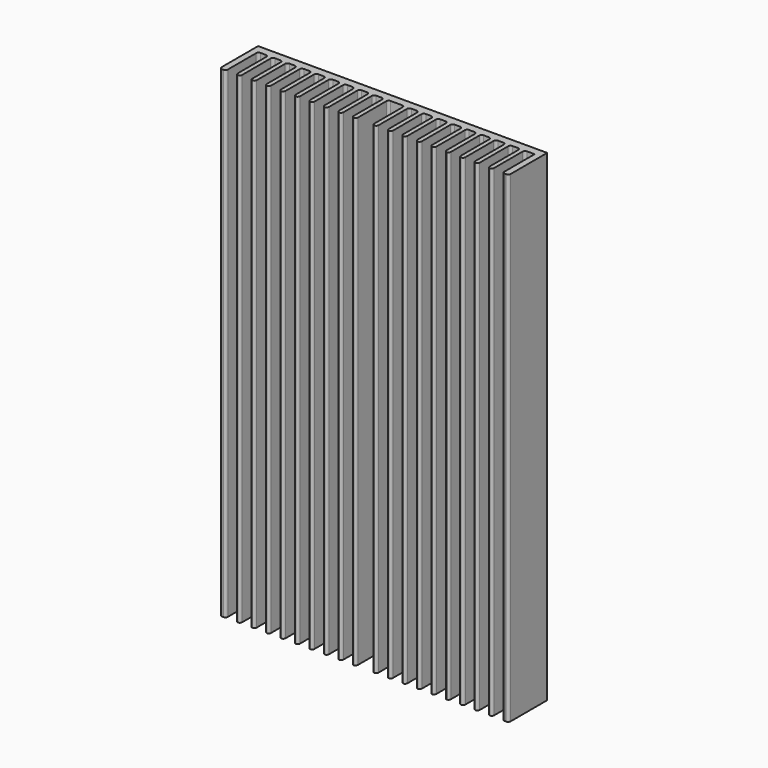
from build123d import *

# Parameters (mm, degrees)
F0_W        = 60
F0_H        = 100
F1_DEPTH    = 10
F2_W        = 2.0929928869
F2_H        = 8.3745439677
F2_W_2      = 1.2923884243
F2_W_3      = 0.8006044626
F3_DEPTH    = 100.001
F4_T1_DEPTH = 100
F4_T3_DEPTH = 102.5


# Not quite as in the source:
# - a fillet or chamfer that OpenCascade refuses, or shapes differently, is made with other operations: its cross-section is extruded or revolved along the edge and cut away or added


with BuildPart() as f1:
    # F0 (on Front) → F1 (new body)
    with BuildSketch(Plane.XZ):
        Rectangle(F0_W, F0_H)
    extrude(amount=F1_DEPTH)

    # F2 (on face) → F3 (cut, through all)
    with BuildSketch(Plane(origin=(0, 0, -50), x_dir=(1, 0, 0), z_dir=(0, 0, -1))):
        with Locations((-27.6461942121, 5.8127280162)):
            Rectangle(F2_W, F2_H)
        with Locations((-24.6461942121, 5.8127280162)):
            Rectangle(F2_W, F2_H)
        with Locations((-21.6461942121, 5.8127280162)):
            Rectangle(F2_W, F2_H)
        with Locations((27.6461942121, 5.8127280162)):
            Rectangle(F2_W, F2_H)
        with Locations((-18.6461942121, 5.8127280162)):
            Rectangle(F2_W, F2_H)
        with Locations((24.6461942121, 5.8127280162)):
            Rectangle(F2_W, F2_H)
        with Locations((-15.6461942121, 5.8127280162)):
            Rectangle(F2_W, F2_H)
        with Locations((21.6461942121, 5.8127280162)):
            Rectangle(F2_W, F2_H)
        with Locations((-12.6461942121, 5.8127280162)):
            Rectangle(F2_W, F2_H)
        with Locations((18.6461942121, 5.8127280162)):
            Rectangle(F2_W, F2_H)
        with Locations((-9.6461942121, 5.8127280162)):
            Rectangle(F2_W, F2_H)
        with Locations((15.6461942121, 5.8127280162)):
            Rectangle(F2_W, F2_H)
        with Locations((-6.6461942121, 5.8127280162)):
            Rectangle(F2_W, F2_H)
        with Locations((12.6461942121, 5.8127280162)):
            Rectangle(F2_W, F2_H)
        with Locations((-3.6461942121, 5.8127280162)):
            Rectangle(F2_W, F2_H)
        with Locations((9.6461942121, 5.8127280162)):
            Rectangle(F2_W, F2_H)
        with Locations((-1.0464964435, 5.8127280162)):
            Rectangle(F2_W_2, F2_H)
        with Locations((0, 5.8127280162)):
            Rectangle(F2_W_3, F2_H)
        with Locations((6.6461942121, 5.8127280162)):
            Rectangle(F2_W, F2_H)
        with Locations((1.0464964435, 5.8127280162)):
            Rectangle(F2_W_2, F2_H)
        with Locations((3.6461942121, 5.8127280162)):
            Rectangle(F2_W, F2_H)
    extrude(amount=-F3_DEPTH, mode=Mode.SUBTRACT)

    # F4: fillet of radius 0.5 on 77 edges, made by hand

    # F4_s2 → F4_t1 (join)
    with BuildSketch(Plane.XY.offset(-50)):
        with BuildLine():
            ThreePointArc((-28.1926906556, -1.6254560323), (-28.5462440462, -1.7719026417), (-28.6926906556, -2.1254560323))
            Line((-28.6926906556, -2.1254560323), (-28.6926906556, -1.6254560323))
            Line((-28.6926906556, -1.6254560323), (-28.1926906556, -1.6254560323))
        make_face()
        with BuildLine():
            ThreePointArc((-26.5996977687, -2.1254560323), (-26.7461443781, -1.7719026417), (-27.0996977687, -1.6254560323))
            Line((-27.0996977687, -1.6254560323), (-26.5996977687, -1.6254560323))
            Line((-26.5996977687, -1.6254560323), (-26.5996977687, -2.1254560323))
        make_face()
        with BuildLine():
            ThreePointArc((-25.1926906556, -1.6254560323), (-25.5462440462, -1.7719026417), (-25.6926906556, -2.1254560323))
            Line((-25.6926906556, -2.1254560323), (-25.6926906556, -1.6254560323))
            Line((-25.6926906556, -1.6254560323), (-25.1926906556, -1.6254560323))
        make_face()
        with BuildLine():
            ThreePointArc((-22.1926906556, -1.6254560323), (-22.5462440462, -1.7719026417), (-22.6926906556, -2.1254560323))
            Line((-22.6926906556, -2.1254560323), (-22.6926906556, -1.6254560323))
            Line((-22.6926906556, -1.6254560323), (-22.1926906556, -1.6254560323))
        make_face()
        with BuildLine():
            ThreePointArc((-19.1926906556, -1.6254560323), (-19.5462440462, -1.7719026417), (-19.6926906556, -2.1254560323))
            Line((-19.6926906556, -2.1254560323), (-19.6926906556, -1.6254560323))
            Line((-19.6926906556, -1.6254560323), (-19.1926906556, -1.6254560323))
        make_face()
        with BuildLine():
            ThreePointArc((-16.1926906556, -1.6254560323), (-16.5462440462, -1.7719026417), (-16.6926906556, -2.1254560323))
            Line((-16.6926906556, -2.1254560323), (-16.6926906556, -1.6254560323))
            Line((-16.6926906556, -1.6254560323), (-16.1926906556, -1.6254560323))
        make_face()
        with BuildLine():
            ThreePointArc((-13.1926906556, -1.6254560323), (-13.5462440462, -1.7719026417), (-13.6926906556, -2.1254560323))
            Line((-13.6926906556, -2.1254560323), (-13.6926906556, -1.6254560323))
            Line((-13.6926906556, -1.6254560323), (-13.1926906556, -1.6254560323))
        make_face()
        with BuildLine():
            ThreePointArc((-10.1926906556, -1.6254560323), (-10.5462440462, -1.7719026417), (-10.6926906556, -2.1254560323))
            Line((-10.6926906556, -2.1254560323), (-10.6926906556, -1.6254560323))
            Line((-10.6926906556, -1.6254560323), (-10.1926906556, -1.6254560323))
        make_face()
        with BuildLine():
            ThreePointArc((-7.1926906556, -1.6254560323), (-7.5462440462, -1.7719026417), (-7.6926906556, -2.1254560323))
            Line((-7.6926906556, -2.1254560323), (-7.6926906556, -1.6254560323))
            Line((-7.6926906556, -1.6254560323), (-7.1926906556, -1.6254560323))
        make_face()
        with BuildLine():
            ThreePointArc((-4.1926906556, -1.6254560323), (-4.5462440462, -1.7719026417), (-4.6926906556, -2.1254560323))
            Line((-4.6926906556, -2.1254560323), (-4.6926906556, -1.6254560323))
            Line((-4.6926906556, -1.6254560323), (-4.1926906556, -1.6254560323))
        make_face()
        with BuildLine():
            ThreePointArc((-1.1926906556, -1.6254560323), (-1.5462440462, -1.7719026417), (-1.6926906556, -2.1254560323))
            Line((-1.6926906556, -2.1254560323), (-1.6926906556, -1.6254560323))
            Line((-1.6926906556, -1.6254560323), (-1.1926906556, -1.6254560323))
        make_face()
        with BuildLine():
            ThreePointArc((3.0996977687, -1.6254560323), (2.7461443781, -1.7719026417), (2.5996977687, -2.1254560323))
            Line((2.5996977687, -2.1254560323), (2.5996977687, -1.6254560323))
            Line((2.5996977687, -1.6254560323), (3.0996977687, -1.6254560323))
        make_face()
        with BuildLine():
            ThreePointArc((6.0996977687, -1.6254560323), (5.7461443781, -1.7719026417), (5.5996977687, -2.1254560323))
            Line((5.5996977687, -2.1254560323), (5.5996977687, -1.6254560323))
            Line((5.5996977687, -1.6254560323), (6.0996977687, -1.6254560323))
        make_face()
        with BuildLine():
            ThreePointArc((9.0996977687, -1.6254560323), (8.7461443781, -1.7719026417), (8.5996977687, -2.1254560323))
            Line((8.5996977687, -2.1254560323), (8.5996977687, -1.6254560323))
            Line((8.5996977687, -1.6254560323), (9.0996977687, -1.6254560323))
        make_face()
        with BuildLine():
            ThreePointArc((12.0996977687, -1.6254560323), (11.7461443781, -1.7719026417), (11.5996977687, -2.1254560323))
            Line((11.5996977687, -2.1254560323), (11.5996977687, -1.6254560323))
            Line((11.5996977687, -1.6254560323), (12.0996977687, -1.6254560323))
        make_face()
        with BuildLine():
            ThreePointArc((15.0996977687, -1.6254560323), (14.7461443781, -1.7719026417), (14.5996977687, -2.1254560323))
            Line((14.5996977687, -2.1254560323), (14.5996977687, -1.6254560323))
            Line((14.5996977687, -1.6254560323), (15.0996977687, -1.6254560323))
        make_face()
        with BuildLine():
            ThreePointArc((18.0996977687, -1.6254560323), (17.7461443781, -1.7719026417), (17.5996977687, -2.1254560323))
            Line((17.5996977687, -2.1254560323), (17.5996977687, -1.6254560323))
            Line((17.5996977687, -1.6254560323), (18.0996977687, -1.6254560323))
        make_face()
        with BuildLine():
            ThreePointArc((21.0996977687, -1.6254560323), (20.7461443781, -1.7719026417), (20.5996977687, -2.1254560323))
            Line((20.5996977687, -2.1254560323), (20.5996977687, -1.6254560323))
            Line((20.5996977687, -1.6254560323), (21.0996977687, -1.6254560323))
        make_face()
        with BuildLine():
            ThreePointArc((24.0996977687, -1.6254560323), (23.7461443781, -1.7719026417), (23.5996977687, -2.1254560323))
            Line((23.5996977687, -2.1254560323), (23.5996977687, -1.6254560323))
            Line((23.5996977687, -1.6254560323), (24.0996977687, -1.6254560323))
        make_face()
        with BuildLine():
            ThreePointArc((27.0996977687, -1.6254560323), (26.7461443781, -1.7719026417), (26.5996977687, -2.1254560323))
            Line((26.5996977687, -2.1254560323), (26.5996977687, -1.6254560323))
            Line((26.5996977687, -1.6254560323), (27.0996977687, -1.6254560323))
        make_face()
        with BuildLine():
            ThreePointArc((-23.5996977687, -2.1254560323), (-23.7461443781, -1.7719026417), (-24.0996977687, -1.6254560323))
            Line((-24.0996977687, -1.6254560323), (-23.5996977687, -1.6254560323))
            Line((-23.5996977687, -1.6254560323), (-23.5996977687, -2.1254560323))
        make_face()
        with BuildLine():
            ThreePointArc((-20.5996977687, -2.1254560323), (-20.7461443781, -1.7719026417), (-21.0996977687, -1.6254560323))
            Line((-21.0996977687, -1.6254560323), (-20.5996977687, -1.6254560323))
            Line((-20.5996977687, -1.6254560323), (-20.5996977687, -2.1254560323))
        make_face()
        with BuildLine():
            ThreePointArc((-17.5996977687, -2.1254560323), (-17.7461443781, -1.7719026417), (-18.0996977687, -1.6254560323))
            Line((-18.0996977687, -1.6254560323), (-17.5996977687, -1.6254560323))
            Line((-17.5996977687, -1.6254560323), (-17.5996977687, -2.1254560323))
        make_face()
        with BuildLine():
            ThreePointArc((-14.5996977687, -2.1254560323), (-14.7461443781, -1.7719026417), (-15.0996977687, -1.6254560323))
            Line((-15.0996977687, -1.6254560323), (-14.5996977687, -1.6254560323))
            Line((-14.5996977687, -1.6254560323), (-14.5996977687, -2.1254560323))
        make_face()
        with BuildLine():
            ThreePointArc((-11.5996977687, -2.1254560323), (-11.7461443781, -1.7719026417), (-12.0996977687, -1.6254560323))
            Line((-12.0996977687, -1.6254560323), (-11.5996977687, -1.6254560323))
            Line((-11.5996977687, -1.6254560323), (-11.5996977687, -2.1254560323))
        make_face()
        with BuildLine():
            ThreePointArc((-8.5996977687, -2.1254560323), (-8.7461443781, -1.7719026417), (-9.0996977687, -1.6254560323))
            Line((-9.0996977687, -1.6254560323), (-8.5996977687, -1.6254560323))
            Line((-8.5996977687, -1.6254560323), (-8.5996977687, -2.1254560323))
        make_face()
        with BuildLine():
            ThreePointArc((-5.5996977687, -2.1254560323), (-5.7461443781, -1.7719026417), (-6.0996977687, -1.6254560323))
            Line((-6.0996977687, -1.6254560323), (-5.5996977687, -1.6254560323))
            Line((-5.5996977687, -1.6254560323), (-5.5996977687, -2.1254560323))
        make_face()
        with BuildLine():
            ThreePointArc((-2.5996977687, -2.1254560323), (-2.7461443781, -1.7719026417), (-3.0996977687, -1.6254560323))
            Line((-3.0996977687, -1.6254560323), (-2.5996977687, -1.6254560323))
            Line((-2.5996977687, -1.6254560323), (-2.5996977687, -2.1254560323))
        make_face()
        with BuildLine():
            ThreePointArc((1.6926906556, -2.1254560323), (1.5462440462, -1.7719026417), (1.1926906556, -1.6254560323))
            Line((1.1926906556, -1.6254560323), (1.6926906556, -1.6254560323))
            Line((1.6926906556, -1.6254560323), (1.6926906556, -2.1254560323))
        make_face()
        with BuildLine():
            ThreePointArc((4.6926906556, -2.1254560323), (4.5462440462, -1.7719026417), (4.1926906556, -1.6254560323))
            Line((4.1926906556, -1.6254560323), (4.6926906556, -1.6254560323))
            Line((4.6926906556, -1.6254560323), (4.6926906556, -2.1254560323))
        make_face()
        with BuildLine():
            ThreePointArc((7.6926906556, -2.1254560323), (7.5462440462, -1.7719026417), (7.1926906556, -1.6254560323))
            Line((7.1926906556, -1.6254560323), (7.6926906556, -1.6254560323))
            Line((7.6926906556, -1.6254560323), (7.6926906556, -2.1254560323))
        make_face()
        with BuildLine():
            ThreePointArc((10.6926906556, -2.1254560323), (10.5462440462, -1.7719026417), (10.1926906556, -1.6254560323))
            Line((10.1926906556, -1.6254560323), (10.6926906556, -1.6254560323))
            Line((10.6926906556, -1.6254560323), (10.6926906556, -2.1254560323))
        make_face()
        with BuildLine():
            ThreePointArc((13.6926906556, -2.1254560323), (13.5462440462, -1.7719026417), (13.1926906556, -1.6254560323))
            Line((13.1926906556, -1.6254560323), (13.6926906556, -1.6254560323))
            Line((13.6926906556, -1.6254560323), (13.6926906556, -2.1254560323))
        make_face()
        with BuildLine():
            ThreePointArc((16.6926906556, -2.1254560323), (16.5462440462, -1.7719026417), (16.1926906556, -1.6254560323))
            Line((16.1926906556, -1.6254560323), (16.6926906556, -1.6254560323))
            Line((16.6926906556, -1.6254560323), (16.6926906556, -2.1254560323))
        make_face()
        with BuildLine():
            ThreePointArc((19.6926906556, -2.1254560323), (19.5462440462, -1.7719026417), (19.1926906556, -1.6254560323))
            Line((19.1926906556, -1.6254560323), (19.6926906556, -1.6254560323))
            Line((19.6926906556, -1.6254560323), (19.6926906556, -2.1254560323))
        make_face()
        with BuildLine():
            ThreePointArc((22.6926906556, -2.1254560323), (22.5462440462, -1.7719026417), (22.1926906556, -1.6254560323))
            Line((22.1926906556, -1.6254560323), (22.6926906556, -1.6254560323))
            Line((22.6926906556, -1.6254560323), (22.6926906556, -2.1254560323))
        make_face()
        with BuildLine():
            ThreePointArc((25.6926906556, -2.1254560323), (25.5462440462, -1.7719026417), (25.1926906556, -1.6254560323))
            Line((25.1926906556, -1.6254560323), (25.6926906556, -1.6254560323))
            Line((25.6926906556, -1.6254560323), (25.6926906556, -2.1254560323))
        make_face()
    extrude(amount=F4_T1_DEPTH)

    # F4_s4 → F4_t3 (cut)
    with BuildSketch(Plane.XY.offset(-51.25)):
        with BuildLine():
            ThreePointArc((-28.6926906556, -9.5), (-28.839137265, -9.8535533906), (-29.1926906556, -10))
            Line((-29.1926906556, -10), (-28.6926906556, -10))
            Line((-28.6926906556, -10), (-28.6926906556, -9.5))
        make_face()
        with BuildLine():
            ThreePointArc((-26.0996977687, -10), (-26.4532511593, -9.8535533906), (-26.5996977687, -9.5))
            Line((-26.5996977687, -9.5), (-26.5996977687, -10))
            Line((-26.5996977687, -10), (-26.0996977687, -10))
        make_face()
        with BuildLine():
            ThreePointArc((-25.6926906556, -9.5), (-25.839137265, -9.8535533906), (-26.1926906556, -10))
            Line((-26.1926906556, -10), (-25.6926906556, -10))
            Line((-25.6926906556, -10), (-25.6926906556, -9.5))
        make_face()
        with BuildLine():
            ThreePointArc((-22.6926906556, -9.5), (-22.839137265, -9.8535533906), (-23.1926906556, -10))
            Line((-23.1926906556, -10), (-22.6926906556, -10))
            Line((-22.6926906556, -10), (-22.6926906556, -9.5))
        make_face()
        with BuildLine():
            ThreePointArc((-19.6926906556, -9.5), (-19.839137265, -9.8535533906), (-20.1926906556, -10))
            Line((-20.1926906556, -10), (-19.6926906556, -10))
            Line((-19.6926906556, -10), (-19.6926906556, -9.5))
        make_face()
        with BuildLine():
            ThreePointArc((-16.6926906556, -9.5), (-16.839137265, -9.8535533906), (-17.1926906556, -10))
            Line((-17.1926906556, -10), (-16.6926906556, -10))
            Line((-16.6926906556, -10), (-16.6926906556, -9.5))
        make_face()
        with BuildLine():
            ThreePointArc((-13.6926906556, -9.5), (-13.839137265, -9.8535533906), (-14.1926906556, -10))
            Line((-14.1926906556, -10), (-13.6926906556, -10))
            Line((-13.6926906556, -10), (-13.6926906556, -9.5))
        make_face()
        with BuildLine():
            ThreePointArc((-10.6926906556, -9.5), (-10.839137265, -9.8535533906), (-11.1926906556, -10))
            Line((-11.1926906556, -10), (-10.6926906556, -10))
            Line((-10.6926906556, -10), (-10.6926906556, -9.5))
        make_face()
        with BuildLine():
            ThreePointArc((-7.6926906556, -9.5), (-7.839137265, -9.8535533906), (-8.1926906556, -10))
            Line((-8.1926906556, -10), (-7.6926906556, -10))
            Line((-7.6926906556, -10), (-7.6926906556, -9.5))
        make_face()
        with BuildLine():
            ThreePointArc((-4.6926906556, -9.5), (-4.839137265, -9.8535533906), (-5.1926906556, -10))
            Line((-5.1926906556, -10), (-4.6926906556, -10))
            Line((-4.6926906556, -10), (-4.6926906556, -9.5))
        make_face()
        with BuildLine():
            ThreePointArc((-1.6926906556, -9.5), (-1.839137265, -9.8535533906), (-2.1926906556, -10))
            Line((-2.1926906556, -10), (-1.6926906556, -10))
            Line((-1.6926906556, -10), (-1.6926906556, -9.5))
        make_face()
        with BuildLine():
            ThreePointArc((2.5996977687, -9.5), (2.4532511593, -9.8535533906), (2.0996977687, -10))
            Line((2.0996977687, -10), (2.5996977687, -10))
            Line((2.5996977687, -10), (2.5996977687, -9.5))
        make_face()
        with BuildLine():
            ThreePointArc((5.5996977687, -9.5), (5.4532511593, -9.8535533906), (5.0996977687, -10))
            Line((5.0996977687, -10), (5.5996977687, -10))
            Line((5.5996977687, -10), (5.5996977687, -9.5))
        make_face()
        with BuildLine():
            ThreePointArc((8.5996977687, -9.5), (8.4532511593, -9.8535533906), (8.0996977687, -10))
            Line((8.0996977687, -10), (8.5996977687, -10))
            Line((8.5996977687, -10), (8.5996977687, -9.5))
        make_face()
        with BuildLine():
            ThreePointArc((11.5996977687, -9.5), (11.4532511593, -9.8535533906), (11.0996977687, -10))
            Line((11.0996977687, -10), (11.5996977687, -10))
            Line((11.5996977687, -10), (11.5996977687, -9.5))
        make_face()
        with BuildLine():
            ThreePointArc((14.5996977687, -9.5), (14.4532511593, -9.8535533906), (14.0996977687, -10))
            Line((14.0996977687, -10), (14.5996977687, -10))
            Line((14.5996977687, -10), (14.5996977687, -9.5))
        make_face()
        with BuildLine():
            ThreePointArc((17.5996977687, -9.5), (17.4532511593, -9.8535533906), (17.0996977687, -10))
            Line((17.0996977687, -10), (17.5996977687, -10))
            Line((17.5996977687, -10), (17.5996977687, -9.5))
        make_face()
        with BuildLine():
            ThreePointArc((20.5996977687, -9.5), (20.4532511593, -9.8535533906), (20.0996977687, -10))
            Line((20.0996977687, -10), (20.5996977687, -10))
            Line((20.5996977687, -10), (20.5996977687, -9.5))
        make_face()
        with BuildLine():
            ThreePointArc((23.5996977687, -9.5), (23.4532511593, -9.8535533906), (23.0996977687, -10))
            Line((23.0996977687, -10), (23.5996977687, -10))
            Line((23.5996977687, -10), (23.5996977687, -9.5))
        make_face()
        with BuildLine():
            ThreePointArc((26.5996977687, -9.5), (26.4532511593, -9.8535533906), (26.0996977687, -10))
            Line((26.0996977687, -10), (26.5996977687, -10))
            Line((26.5996977687, -10), (26.5996977687, -9.5))
        make_face()
        with BuildLine():
            ThreePointArc((29.1926906556, -10), (28.839137265, -9.8535533906), (28.6926906556, -9.5))
            Line((28.6926906556, -9.5), (28.6926906556, -10))
            Line((28.6926906556, -10), (29.1926906556, -10))
        make_face()
        with BuildLine():
            ThreePointArc((30, -9.5), (29.8535533906, -9.8535533906), (29.5, -10))
            Line((29.5, -10), (30, -10))
            Line((30, -10), (30, -9.5))
        make_face()
        with BuildLine():
            ThreePointArc((-29.5, -10), (-29.8535533906, -9.8535533906), (-30, -9.5))
            Line((-30, -9.5), (-30, -10))
            Line((-30, -10), (-29.5, -10))
        make_face()
        with BuildLine():
            ThreePointArc((-23.0996977687, -10), (-23.4532511593, -9.8535533906), (-23.5996977687, -9.5))
            Line((-23.5996977687, -9.5), (-23.5996977687, -10))
            Line((-23.5996977687, -10), (-23.0996977687, -10))
        make_face()
        with BuildLine():
            ThreePointArc((-20.0996977687, -10), (-20.4532511593, -9.8535533906), (-20.5996977687, -9.5))
            Line((-20.5996977687, -9.5), (-20.5996977687, -10))
            Line((-20.5996977687, -10), (-20.0996977687, -10))
        make_face()
        with BuildLine():
            ThreePointArc((-17.0996977687, -10), (-17.4532511593, -9.8535533906), (-17.5996977687, -9.5))
            Line((-17.5996977687, -9.5), (-17.5996977687, -10))
            Line((-17.5996977687, -10), (-17.0996977687, -10))
        make_face()
        with BuildLine():
            ThreePointArc((-14.0996977687, -10), (-14.4532511593, -9.8535533906), (-14.5996977687, -9.5))
            Line((-14.5996977687, -9.5), (-14.5996977687, -10))
            Line((-14.5996977687, -10), (-14.0996977687, -10))
        make_face()
        with BuildLine():
            ThreePointArc((-11.0996977687, -10), (-11.4532511593, -9.8535533906), (-11.5996977687, -9.5))
            Line((-11.5996977687, -9.5), (-11.5996977687, -10))
            Line((-11.5996977687, -10), (-11.0996977687, -10))
        make_face()
        with BuildLine():
            ThreePointArc((-8.0996977687, -10), (-8.4532511593, -9.8535533906), (-8.5996977687, -9.5))
            Line((-8.5996977687, -9.5), (-8.5996977687, -10))
            Line((-8.5996977687, -10), (-8.0996977687, -10))
        make_face()
        with BuildLine():
            ThreePointArc((-5.0996977687, -10), (-5.4532511593, -9.8535533906), (-5.5996977687, -9.5))
            Line((-5.5996977687, -9.5), (-5.5996977687, -10))
            Line((-5.5996977687, -10), (-5.0996977687, -10))
        make_face()
        with BuildLine():
            ThreePointArc((-2.0996977687, -10), (-2.4532511593, -9.8535533906), (-2.5996977687, -9.5))
            Line((-2.5996977687, -9.5), (-2.5996977687, -10))
            Line((-2.5996977687, -10), (-2.0996977687, -10))
        make_face()
        with BuildLine():
            ThreePointArc((2.1926906556, -10), (1.839137265, -9.8535533906), (1.6926906556, -9.5))
            Line((1.6926906556, -9.5), (1.6926906556, -10))
            Line((1.6926906556, -10), (2.1926906556, -10))
        make_face()
        with BuildLine():
            ThreePointArc((5.1926906556, -10), (4.839137265, -9.8535533906), (4.6926906556, -9.5))
            Line((4.6926906556, -9.5), (4.6926906556, -10))
            Line((4.6926906556, -10), (5.1926906556, -10))
        make_face()
        with BuildLine():
            ThreePointArc((8.1926906556, -10), (7.839137265, -9.8535533906), (7.6926906556, -9.5))
            Line((7.6926906556, -9.5), (7.6926906556, -10))
            Line((7.6926906556, -10), (8.1926906556, -10))
        make_face()
        with BuildLine():
            ThreePointArc((11.1926906556, -10), (10.839137265, -9.8535533906), (10.6926906556, -9.5))
            Line((10.6926906556, -9.5), (10.6926906556, -10))
            Line((10.6926906556, -10), (11.1926906556, -10))
        make_face()
        with BuildLine():
            ThreePointArc((14.1926906556, -10), (13.839137265, -9.8535533906), (13.6926906556, -9.5))
            Line((13.6926906556, -9.5), (13.6926906556, -10))
            Line((13.6926906556, -10), (14.1926906556, -10))
        make_face()
        with BuildLine():
            ThreePointArc((17.1926906556, -10), (16.839137265, -9.8535533906), (16.6926906556, -9.5))
            Line((16.6926906556, -9.5), (16.6926906556, -10))
            Line((16.6926906556, -10), (17.1926906556, -10))
        make_face()
        with BuildLine():
            ThreePointArc((20.1926906556, -10), (19.839137265, -9.8535533906), (19.6926906556, -9.5))
            Line((19.6926906556, -9.5), (19.6926906556, -10))
            Line((19.6926906556, -10), (20.1926906556, -10))
        make_face()
        with BuildLine():
            ThreePointArc((23.1926906556, -10), (22.839137265, -9.8535533906), (22.6926906556, -9.5))
            Line((22.6926906556, -9.5), (22.6926906556, -10))
            Line((22.6926906556, -10), (23.1926906556, -10))
        make_face()
        with BuildLine():
            ThreePointArc((26.1926906556, -10), (25.839137265, -9.8535533906), (25.6926906556, -9.5))
            Line((25.6926906556, -9.5), (25.6926906556, -10))
            Line((25.6926906556, -10), (26.1926906556, -10))
        make_face()
    extrude(amount=F4_T3_DEPTH, mode=Mode.SUBTRACT)


solid = f1.part
